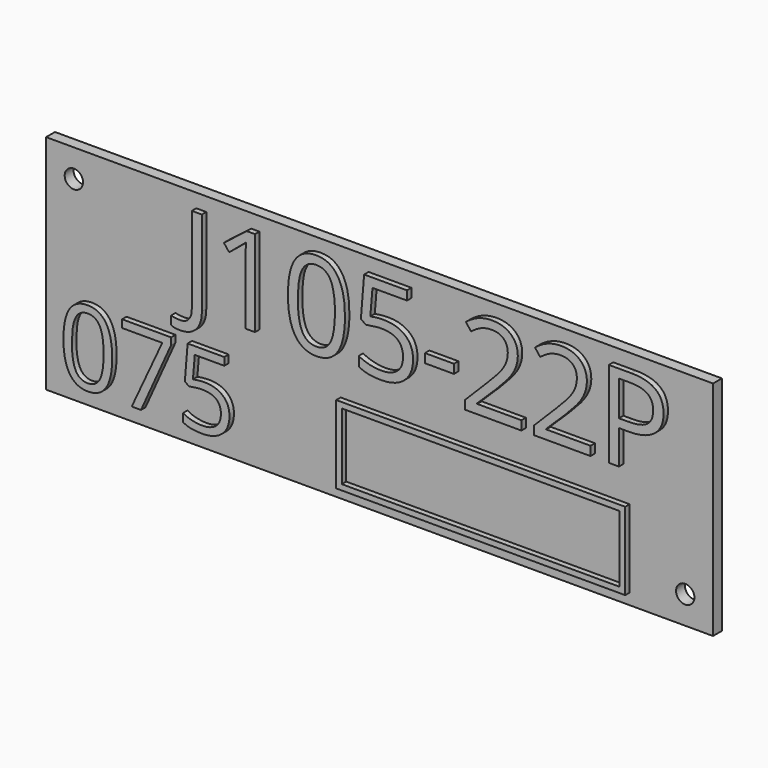
from build123d import *

# Parameters (mm, degrees)
F0_W         = 120
F0_H         = 40
F1_DEPTH     = 2
F3_D         = 3.3
F4_TEXT_SIZE = 21.733388673
F5_DEPTH     = 1
F6_TEXT_SIZE = 18.5776487663
F7_DEPTH     = 1
F8_W         = 52
F8_H         = 14
F8_W_2       = 49.99999962
F8_H_2       = 11.99999962
F9_DEPTH     = 1


# Not quite as in the source:
# - Text() gives the source's letters only with a copy of the font that has no kerning and outlines rounded to 1/6400 em; it was checked with that copy


with BuildPart() as f1:
    # F0 (on Front) → F1 (new body)
    with BuildSketch(Plane.XZ):
        Rectangle(F0_W, F0_H)
    extrude(amount=F1_DEPTH)

    # F3 (through all)
    with Locations(Plane.XZ.offset(2)):
        with Locations((-55, 15), (55, -15)):
            Hole(F3_D / 2)

    # F4 (on face) → F5 (join)
    with BuildSketch(Plane.XZ.offset(2)):
        with Locations((-35, 2)):
            Text('J105-22P', F4_TEXT_SIZE, font='Open Sans', text_align=(TextAlign.LEFT, TextAlign.BOTTOM))
    extrude(amount=F5_DEPTH)

    # F6 (on face) → F7 (join)
    with BuildSketch(Plane.XZ.offset(2)):
        with Locations((-57, -17)):
            Text('075', F6_TEXT_SIZE, font='Open Sans', text_align=(TextAlign.LEFT, TextAlign.BOTTOM))
    extrude(amount=F7_DEPTH)

    # F8 (on face) → F9 (join)
    with BuildSketch(Plane.XZ.offset(2)):
        with Locations((19, -11)):
            Rectangle(F8_W, F8_H)
        with Locations((19, -11)):
            Rectangle(F8_W_2, F8_H_2, mode=Mode.SUBTRACT)
    extrude(amount=F9_DEPTH)


solid = f1.part
